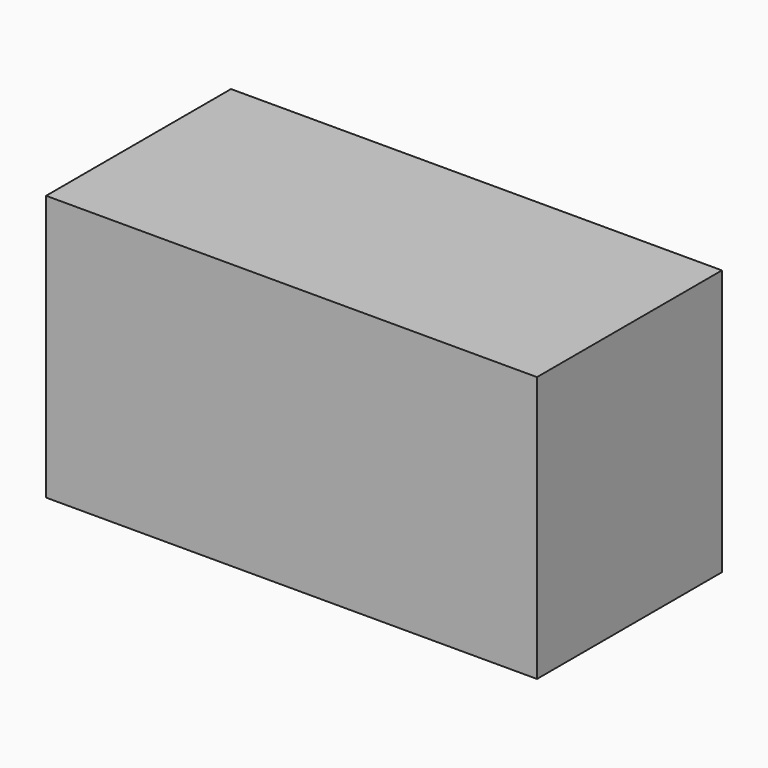
from build123d import *

# Parameters (mm, degrees)
F0_W     = 107.8889481723
F0_H     = 58.4026928991
F1_DEPTH = 50.8


# Not quite as in the source:
# - a feature of the source that left no trace in its solid (it failed there, or was rolled back) is left out


with BuildPart() as f1:
    # F0 (on Front) → F1 (new body)
    with BuildSketch(Plane.XZ):
        with Locations((2.45202519, 0.6687296554)):
            Rectangle(F0_W, F0_H)
    extrude(amount=F1_DEPTH)


solid = f1.part
